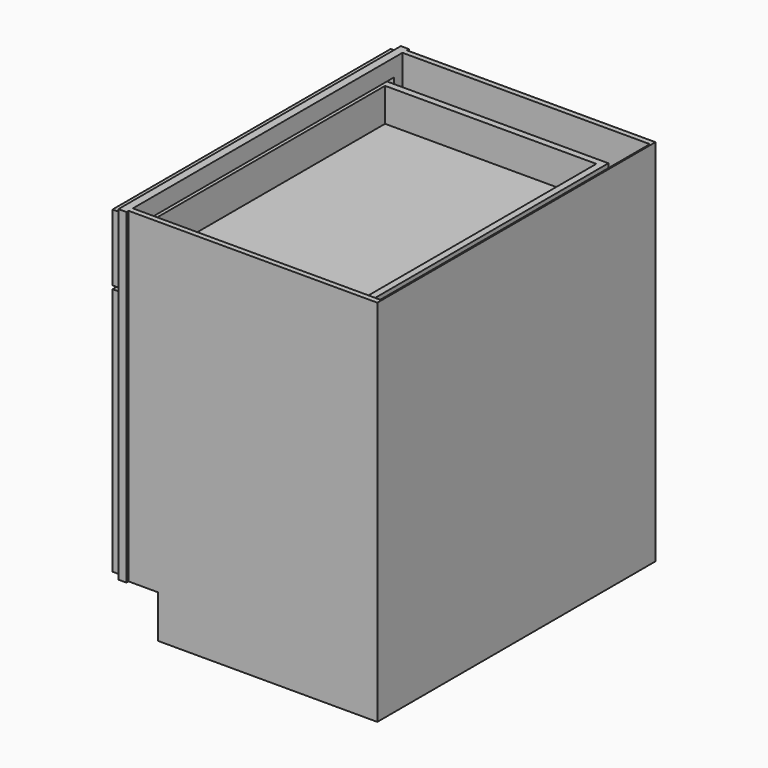
from build123d import *

# Parameters (mm, degrees)
F0_W          = 609.6
F0_H          = 876.3
F1_DEPTH      = 838.2
F2_W          = 88.9
F2_H          = 101.6
F3_DEPTH      = 838.201
F4_W          = 748.8836065574
F4_H          = 692.15
F5_DEPTH      = 19.05
F6_W          = 590.55
F6_H          = 6.35
F7_DEPTH      = 876.301
F8_W          = 587.375
F8_H          = 800.1
F9_DEPTH      = 733.425
F10_W         = 748.8836065574
F10_H         = 41.275
F11_DEPTH     = 19.05
F12_W         = 412.75
F12_H         = 590.5627
F12_W_2       = 298.45
F12_H_2       = 476.2627
F13_DEPTH     = 19.05
F14_W         = 6.35
F14_H         = 298.45
F15_DEPTH     = 476.2627
F16_SIZE      = 3.175
F17_W         = 825.5
F17_H         = 158.75
F17_W_2       = 711.2
F17_H_2       = 82.55
F18_DEPTH     = 19.05
F19_W         = 6.35
F19_H         = 711.2
F20_DEPTH     = 82.55
F21_SIZE      = 3.175
F22_W         = 504.825
F22_H         = 800.1
F23_DEPTH     = 101.6
F24_W         = 736.6
F24_H         = 95.25
F25_DEPTH     = 533.4
F26_T         = 15.875
F26_T3_DEPTH  = 37.249261314
F26_T5_DEPTH  = 37.249261314
F26_T7_DEPTH  = 37.249261314
F26_T9_DEPTH  = 37.249261314
F26_T11_DEPTH = 36.5125
F26_T13_DEPTH = 742.95
F26_T15_DEPTH = 114.3
F26_T17_DEPTH = 127
F26_T19_DEPTH = 768.35
F26_T21_DEPTH = 111.125
F26_T23_DEPTH = 36.5125


# Not quite as in the source:
# - a shell that OpenCascade refuses in one call is made with other operations: the cavity is built on its own and cut out


with BuildPart() as f1:
    # F0 (on Front) → F1 (new body)
    with BuildSketch(Plane.XZ):
        Rectangle(F0_W, F0_H)
    extrude(amount=-F1_DEPTH)

    # F2 (on face) → F3 (cut, through all)
    with BuildSketch(Plane.XZ):
        with Locations((-260.35, -387.35)):
            Rectangle(F2_W, F2_H)
    extrude(amount=-F3_DEPTH, mode=Mode.SUBTRACT)

    # F4 (on face) → F5 (cut)
    with BuildSketch(Plane(origin=(-304.8, 0, 0), x_dir=(0, -1, 0), z_dir=(-1, 0, 0))):
        with Locations((-419.1, 50.8)):
            Rectangle(F4_W, F4_H)
    extrude(amount=-F5_DEPTH, mode=Mode.SUBTRACT)

    # F6 (on face) → F7 (cut, through all)
    with BuildSketch(Plane.XY.offset(438.15)):
        with Locations((9.525, 835.025)):
            Rectangle(F6_W, F6_H)
        with Locations((9.525, 3.175)):
            Rectangle(F6_W, F6_H)
    extrude(amount=-F7_DEPTH, mode=Mode.SUBTRACT)

    # F8 (on face) → F9 (cut, through all)
    with BuildSketch(Plane.XY.offset(438.15)):
        with Locations((7.9375, 419.1)):
            Rectangle(F8_W, F8_H)
    extrude(amount=-F9_DEPTH, mode=Mode.SUBTRACT)

    # F10 (on face) → F11 (join, through all)
    with BuildSketch(Plane(origin=(-304.8, 0, 0), x_dir=(0, -1, 0), z_dir=(-1, 0, 0))):
        with Locations((-419.1, 265.1125)):
            Rectangle(F10_W, F10_H)
    extrude(amount=-F11_DEPTH)

    # F22 (on face) → F23 (cut)
    with BuildSketch(Plane(origin=(0, 0, -438.15), x_dir=(1, 0, 0), z_dir=(0, 0, -1))):
        with Locations((49.2125, -419.1)):
            Rectangle(F22_W, F22_H)
    extrude(amount=-F23_DEPTH, mode=Mode.SUBTRACT)


with BuildPart() as f13:
    # F12 (on face) → F13 (new body)
    with BuildSketch(Plane(origin=(-304.8, 0, 0), x_dir=(0, -1, 0), z_dir=(-1, 0, 0))):
        with Locations((-625.475, -33.33115)):
            Rectangle(F12_W, F12_H)
        with Locations((-625.475, -33.33115)):
            Rectangle(F12_W_2, F12_H_2, mode=Mode.SUBTRACT)
    extrude(amount=F13_DEPTH)

    # F14 (on face) → F15 (join, through all)
    with BuildSketch(Plane.XY.offset(-271.4625)):
        with Locations((-312.7375, 625.475)):
            Rectangle(F14_W, F14_H)
    extrude(amount=F15_DEPTH)

    # F16
    f16_edges = [f13.edges().sort_by_distance(p)[0] for p in [
        (-323.85, 774.7, -33.33115),
        (-323.85, 625.475, -271.4625),
        (-323.85, 476.25, -33.33115),
        (-323.85, 625.475, 204.8002),
    ]]
    chamfer(f16_edges, length=F16_SIZE)


with BuildPart() as f18:
    # F17 (on face) → F18 (new body)
    with BuildSketch(Plane(origin=(-304.8, 0, 0), x_dir=(0, -1, 0), z_dir=(-1, 0, 0))):
        with Locations((-419.1, 349.25)):
            Rectangle(F17_W, F17_H)
        with Locations((-419.1, 349.25)):
            Rectangle(F17_W_2, F17_H_2, mode=Mode.SUBTRACT)
    extrude(amount=F18_DEPTH)

    # F19 (on face) → F20 (join, through all)
    with BuildSketch(Plane.XY.offset(307.975)):
        with Locations((-312.7375, 419.1)):
            Rectangle(F19_W, F19_H)
    extrude(amount=F20_DEPTH)

    # F21
    f21_edges = [f18.edges().sort_by_distance(p)[0] for p in [
        (-323.85, 419.1, 307.975),
        (-323.85, 774.7, 349.25),
        (-323.85, 419.1, 390.525),
        (-323.85, 63.5, 349.25),
    ]]
    chamfer(f21_edges, length=F21_SIZE)

    # F24 (on face) → F25 (join)
    with BuildSketch(Plane.YZ.offset(-304.8)):
        with Locations((419.1, 339.725)):
            Rectangle(F24_W, F24_H)
    extrude(amount=F25_DEPTH)

    # F26: shell of thickness 15.875, made by hand


with BuildPart() as f26_core1:
    # F26_t2: copy of F18
    add(f18.part)

    # the walls: a layer under each face that stays
    f26_faces = [f26_core1.faces().sort_by_distance(p)[0] for p in [
        (-323.85, 694.2666666667, 296.3333333333),
        (-322.2625, 419.1, 306.3875),
        (-322.2625, 61.9125, 349.25),
        (-322.2625, 776.2875, 349.25),
        (-322.2625, 419.1, 392.1125),
        (-314.325, 419.1, 428.625),
        (-314.325, 831.85, 349.25),
        (-314.325, 419.1, 269.875),
        (-314.325, 6.35, 349.25),
        (-318.29375, 419.1, 307.975),
        (-318.29375, 63.5, 349.25),
        (-318.29375, 774.7, 349.25),
        (-318.29375, 419.1, 390.525),
        (-304.8, 694.2666666667, 402.1666666667),
        (-315.9125, 419.1, 349.25),
        (-38.1, 787.4, 339.725),
        (-38.1, 419.1, 292.1),
        (-38.1, 50.8, 339.725),
        (-307.18125, 63.5, 349.25),
        (-307.18125, 419.1, 390.525),
        (-307.18125, 774.7, 349.25),
        (-304.8, 419.1, 347.6625),
        (228.6, 419.1, 339.725),
        (-307.18125, 419.1, 307.975),
        (-309.5625, 419.1, 349.25),
    ]]
    thicken(f26_faces, amount=-F26_T, mode=Mode.SUBTRACT)

    # F26_s4 → F26_t3 (cut)
    with BuildSketch(Plane(origin=(4.5928978099, 4.5928978099, 4.5928978099), x_dir=(-0.7071067812, 0.7071067812, 0), z_dir=(0.5773502692, 0.5773502692, 0.5773502692))):
        Polygon((271.8908726623, 356.5892701441), (263.7152476623, 342.7036353262), (255.7777476623, 347.2863530879), (255.7777476623, 356.4517886113), align=None)
    extrude(amount=F26_T3_DEPTH, mode=Mode.SUBTRACT)

    # F26_s6 → F26_t5 (cut)
    with BuildSketch(Plane(origin=(-274.8071021901, 274.80710219, -274.8071021901), x_dir=(0.7071067812, 0.7071067812, 0), z_dir=(0.5773502692, -0.5773502692, 0.5773502692))):
        Polygon((320.8060313282, 698.7829872109), (328.9816563282, 684.897352393), (336.9191563282, 689.4800701547), (336.9191563282, 698.6455056781), align=None)
    extrude(amount=F26_T5_DEPTH, mode=Mode.SUBTRACT)

    # F26_s8 → F26_t7 (cut)
    with BuildSketch(Plane(origin=(-228.2404355234, -228.2404355234, 228.2404355234), x_dir=(-0.7071067812, 0.7071067812, 0), z_dir=(0.5773502692, 0.5773502692, -0.5773502692))):
        Polygon((271.8908726623, 213.7335916339), (255.7777476623, 213.8710731668), (255.7777476623, 223.0365086901), (263.7152476623, 227.6192264518), align=None)
    extrude(amount=F26_T7_DEPTH, mode=Mode.SUBTRACT)

    # F26_s10 → F26_t9 (cut)
    with BuildSketch(Plane(origin=(-507.6404355234, 507.6404355234, 507.6404355234), x_dir=(0.7071067812, 0.7071067812, 0), z_dir=(0.5773502692, -0.5773502692, -0.5773502692))):
        Polygon((320.8060313282, -128.4601254329), (336.9191563282, -128.3226439001), (336.9191563282, -119.1572083767), (328.9816563282, -114.574490615), align=None)
    extrude(amount=F26_T9_DEPTH, mode=Mode.SUBTRACT)

    # F26_s12 → F26_t11 (cut)
    with BuildSketch(Plane.YZ.offset(-336.55)):
        Polygon((774.54125, 308.13375), (774.7, 292.1), (790.575, 292.1), (790.575, 307.975), align=None)
        Polygon((63.65875, 308.13375), (63.5, 292.1), (47.625, 292.1), (47.625, 307.975), align=None)
        Polygon((63.65875, 390.36625), (47.625, 390.525), (47.625, 406.4), (63.5, 406.4), align=None)
        Polygon((774.54125, 390.36625), (790.575, 390.525), (790.575, 406.4), (774.7, 406.4), align=None)
    extrude(amount=F26_T11_DEPTH, mode=Mode.SUBTRACT)

    # F26_s14 → F26_t13 (cut)
    with BuildSketch(Plane.XZ.offset(-790.575)):
        Polygon((-316.07125, 308.13375), (-315.9125, 292.1), (-300.0375, 292.1), (-300.0375, 307.975), align=None)
        Polygon((-316.07125, 390.36625), (-315.9125, 406.4), (-300.0375, 406.4), (-300.0375, 390.525), align=None)
        Polygon((-309.40375, 390.36625), (-309.5625, 406.4), (-325.4375, 406.4), (-325.4375, 390.525), align=None)
        Polygon((-304.95875, 308.13375), (-288.925, 307.975), (-288.925, 292.1), (-304.8, 292.1), align=None)
        Polygon((-309.40375, 308.13375), (-309.5625, 292.1), (-325.4375, 292.1), (-325.4375, 307.975), align=None)
    extrude(amount=F26_T13_DEPTH, mode=Mode.SUBTRACT)

    # F26_s16 → F26_t15 (cut)
    with BuildSketch(Plane.XY.offset(292.1)):
        Polygon((-316.07125, 63.65875), (-315.9125, 47.625), (-300.0375, 47.625), (-300.0375, 63.5), align=None)
        Polygon((-316.07125, 774.54125), (-315.9125, 790.575), (-300.0375, 790.575), (-300.0375, 774.7), align=None)
        Polygon((-309.40375, 63.65875), (-309.5625, 47.625), (-325.4375, 47.625), (-325.4375, 63.5), align=None)
        Polygon((-309.40375, 774.54125), (-309.5625, 790.575), (-325.4375, 790.575), (-325.4375, 774.7), align=None)
    extrude(amount=F26_T15_DEPTH, mode=Mode.SUBTRACT)

    # F26_s18 → F26_t17 (cut)
    with BuildSketch(Plane.XY.offset(276.225)):
        Polygon((-304.64125, 787.55875), (-320.675, 787.4), (-320.675, 771.525), (-304.8, 771.525), align=None)
        Polygon((-304.64125, 50.64125), (-320.675, 50.8), (-320.675, 66.675), (-304.8, 66.675), align=None)
    extrude(amount=F26_T17_DEPTH, mode=Mode.SUBTRACT)

    # F26_s20 → F26_t19 (cut)
    with BuildSketch(Plane.XZ.offset(-803.275)):
        Polygon((-304.64125, 291.94125), (-320.675, 292.1), (-320.675, 307.975), (-304.8, 307.975), align=None)
    extrude(amount=F26_T19_DEPTH, mode=Mode.SUBTRACT)

    # F26_s22 → F26_t21 (cut)
    with BuildSketch(Plane.XY.offset(292.1)):
        Polygon((-304.95875, 63.65875), (-304.8, 47.625), (-288.925, 47.625), (-288.925, 63.5), align=None)
        Polygon((-304.95875, 774.54125), (-304.8, 790.575), (-288.925, 790.575), (-288.925, 774.7), align=None)
    extrude(amount=F26_T21_DEPTH, mode=Mode.SUBTRACT)

    # F26_s24 → F26_t23 (cut)
    with BuildSketch(Plane.YZ.offset(-325.4375)):
        Polygon((63.65875, 308.13375), (47.625, 307.975), (47.625, 292.1), (63.5, 292.1), align=None)
        Polygon((63.65875, 390.36625), (47.625, 390.525), (47.625, 406.4), (63.5, 406.4), align=None)
        Polygon((774.54125, 390.36625), (774.7, 406.4), (790.575, 406.4), (790.575, 390.525), align=None)
        Polygon((774.54125, 308.13375), (790.575, 307.975), (790.575, 292.1), (774.7, 292.1), align=None)
    extrude(amount=F26_T23_DEPTH, mode=Mode.SUBTRACT)


with BuildPart() as f18_1:
    add(f18.part)

    # what is left inside the walls is the cavity
    f26_cavity = [f26_core1.part.solids().sort_by_distance(p)[0] for p in [
        (45.508333, 419.1, 308.13375),
    ]]
    add(f26_cavity, mode=Mode.SUBTRACT)


with BuildPart() as f27_1:
    # F27: instance of F13
    add(f13.part.mirror(Plane(origin=(-314.325, 419.1, -33.33115), x_dir=(1, 0, 0), z_dir=(0, -1, 0))))


solid = Compound([f1.part, f13.part, f18_1.part, f27_1.part])
